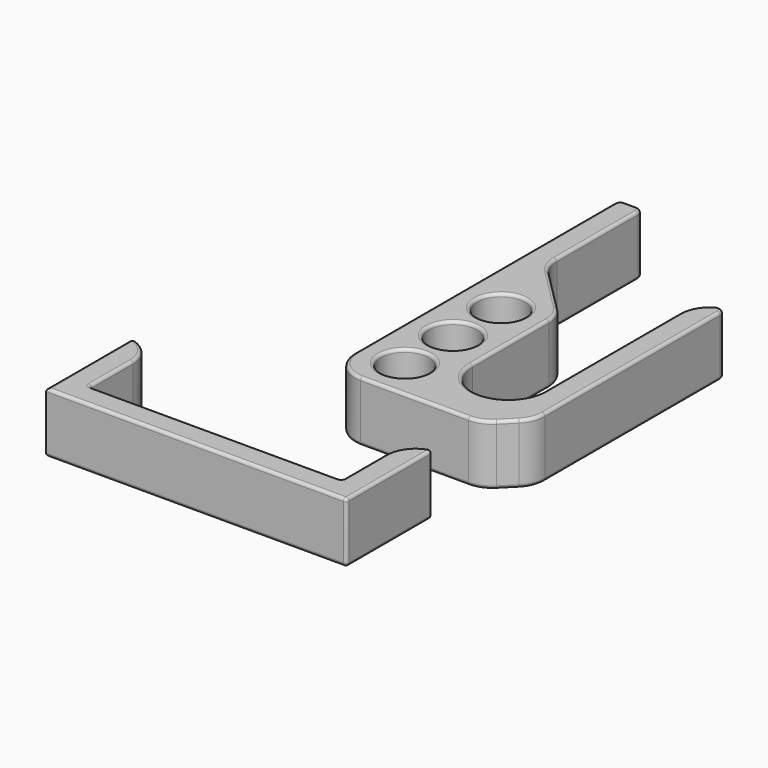
from build123d import *

# Parameters (mm, degrees)
F1_DEPTH     = 10
F2_T1_DEPTH  = 10
F2_T3_DEPTH  = 34.4948974279
F2_T5_DEPTH  = 20.3553390593
F2_T7_DEPTH  = 35
F2_T9_DEPTH  = 20.3553390593
F2_T11_DEPTH = 20.3553390593
F3_R         = 1
F4_R         = 4
F5_DEPTH     = 25
F7_R         = 0.5
F9_DEPTH     = 10
F10_T1_DEPTH = 34.4948974279
F11_R        = 0.5


# Not quite as in the source:
# - a fillet or chamfer that OpenCascade refuses, or shapes differently, is made with other operations: its cross-section is extruded or revolved along the edge and cut away or added
# - a feature names something its author has since deleted; it is built from what else it names


with BuildPart() as f1:
    # F0 (on Top) → F1 (new body)
    with BuildSketch(Plane.XY):
        with BuildLine():
            Line((4, 35.789473919), (0, 35.789473919))
            Line((0, 35.789473919), (0, -24.210526081))
            Line((0, -24.210526081), (25, -24.210526081))
            Line((25, -24.210526081), (30, -19.210526081))
            Line((30, -19.210526081), (30, 20.789473919))
            Line((30, 20.789473919), (26, 20.789473919))
            Line((26, 20.789473919), (26, -12.210526081))
            ThreePointArc((26, -12.210526081), (20, -18.210526081), (14, -12.210526081))
            Line((14, -12.210526081), (14, 5.789473919))
            Line((14, 5.789473919), (4, 15.789473919))
            Line((4, 15.789473919), (4, 35.789473919))
        make_face()
    extrude(amount=F1_DEPTH)

    # F2: fillet of radius 5 on 6 edges, made by hand

    # F2_s2 → F2_t1 (join)
    with BuildSketch(Plane.XY):
        with BuildLine():
            ThreePointArc((5.4644660941, 14.325007825), (4.3806023374, 15.9471245691), (4, 17.8605417309))
            Line((4, 17.8605417309), (4, 15.789473919))
            Line((4, 15.789473919), (5.4644660941, 14.325007825))
        make_face()
    extrude(amount=F2_T1_DEPTH)

    # F2_s4 → F2_t3 (cut)
    with BuildSketch(Plane.XY.offset(-12.2474487139)):
        with BuildLine():
            ThreePointArc((26, 15.8904944335), (27.1270166538, 19.0527720936), (30, 20.789473919))
            Line((30, 20.789473919), (26, 20.789473919))
            Line((26, 20.789473919), (26, 15.8904944335))
        make_face()
    extrude(amount=F2_T3_DEPTH, mode=Mode.SUBTRACT)

    # F2_s6 → F2_t5 (cut)
    with BuildSketch(Plane.XY.offset(-5.1776695297)):
        with BuildLine():
            ThreePointArc((12.5355339059, 7.2539400131), (13.6193976626, 5.631823269), (14, 3.7184061072))
            Line((14, 3.7184061072), (14, 5.789473919))
            Line((14, 5.789473919), (12.5355339059, 7.2539400131))
        make_face()
    extrude(amount=F2_T5_DEPTH, mode=Mode.SUBTRACT)

    # F2_s8 → F2_t7 (cut)
    with BuildSketch(Plane.XY.offset(-12.5)):
        with BuildLine():
            ThreePointArc((5, -24.210526081), (1.4644660941, -22.7460599869), (0, -19.210526081))
            Line((0, -19.210526081), (0, -24.210526081))
            Line((0, -24.210526081), (5, -24.210526081))
        make_face()
    extrude(amount=F2_T7_DEPTH, mode=Mode.SUBTRACT)

    # F2_s10 → F2_t9 (cut)
    with BuildSketch(Plane.XY.offset(-5.1776695297)):
        with BuildLine():
            ThreePointArc((26.4644660941, -22.7460599869), (24.84234935, -23.8299237435), (22.9289321881, -24.210526081))
            Line((22.9289321881, -24.210526081), (25, -24.210526081))
            Line((25, -24.210526081), (26.4644660941, -22.7460599869))
        make_face()
    extrude(amount=F2_T9_DEPTH, mode=Mode.SUBTRACT)

    # F2_s12 → F2_t11 (cut)
    with BuildSketch(Plane.XY.offset(-5.1776695297)):
        with BuildLine():
            ThreePointArc((30, -17.1394582691), (29.6193976626, -19.0528754309), (28.5355339059, -20.674992175))
            Line((28.5355339059, -20.674992175), (30, -19.210526081))
            Line((30, -19.210526081), (30, -17.1394582691))
        make_face()
    extrude(amount=F2_T11_DEPTH, mode=Mode.SUBTRACT)

    # F3
    f3_edges = [f1.edges().sort_by_distance(p)[0] for p in [
        (30, 20.789474, 5),
        (0, 35.789474, 5),
        (4, 35.789474, 5),
    ]]
    fillet(f3_edges, radius=F3_R)


with BuildPart() as f5:
    # F4 (on Top) → F5 (new body)
    with BuildSketch(Plane.XY):
        with Locations((7, 2.5)):
            Circle(F4_R)
    extrude(amount=F5_DEPTH)


with BuildPart() as f5b:
    # F4 (on Top) → F5, piece 2 (new body)
    with BuildSketch(Plane.XY):
        with Locations((7, -7.5)):
            Circle(F4_R)
    extrude(amount=F5_DEPTH)


with BuildPart() as f5c:
    # F4 (on Top) → F5, piece 3 (new body)
    with BuildSketch(Plane.XY):
        with Locations((7, -17.5)):
            Circle(F4_R)
    extrude(amount=F5_DEPTH)


with BuildPart() as f1_1:
    add(f1.part)

    # F6: cut F5c, F5b, F5
    add(f5c.part, mode=Mode.SUBTRACT)
    add(f5b.part, mode=Mode.SUBTRACT)
    add(f5.part, mode=Mode.SUBTRACT)

    # F7
    f7_edges = [f1_1.edges().sort_by_distance(p)[0] for p in [
        (3, -17.5, 10),
        (3, -7.5, 10),
        (3, 2.5, 10),
        (3, 2.5, 0),
        (3, -7.5, 0),
        (3, -17.5, 0),
        (26.669873, 18.390494, 0),
        (29.5, 20.220621, 0),
        (26, 1.839984, 0),
        (30, 1.107569, 0),
        (20, -18.210526, 0),
        (29.619398, -19.052875, 0),
        (14, -4.24606, 0),
        (27.5, -21.710526, 0),
        (13.619398, 5.631823, 0),
        (24.842349, -23.829924, 0),
        (9, 10.789474, 0),
        (13.964466, -24.210526, 0),
        (4.380602, 15.947125, 0),
        (1.464466, -22.74606, 0),
        (4, 26.325008, 0),
        (0, 7.789474, 0),
        (3.707107, 35.496581, 0),
        (0.292893, 35.496581, 0),
        (2, 35.789474, 0),
        (26.669873, 18.390494, 10),
        (29.5, 20.220621, 10),
        (26, 1.839984, 10),
        (30, 1.107569, 10),
        (20, -18.210526, 10),
        (29.619398, -19.052875, 10),
        (14, -4.24606, 10),
        (27.5, -21.710526, 10),
        (13.619398, 5.631823, 10),
        (24.842349, -23.829924, 10),
        (9, 10.789474, 10),
        (13.964466, -24.210526, 10),
        (4.380602, 15.947125, 10),
        (1.464466, -22.74606, 10),
        (4, 26.325008, 10),
        (0, 7.789474, 10),
        (3.707107, 35.496581, 10),
        (0.292893, 35.496581, 10),
        (2, 35.789474, 10),
    ]]
    fillet(f7_edges, radius=F7_R)


with BuildPart() as f9:
    # F8 (on Top) → F9 (new body)
    with BuildSketch(Plane.XY):
        Polygon((-21, -34.1406405903), (-25, -34.1406405903), (-25, -52.1406405903), (25, -52.1406405903), (25, -34.1406405903), (21, -34.1406405903), (21, -48.1406405903), (-21, -48.1406405903), align=None)
    extrude(amount=F9_DEPTH)

    # F10: fillet of radius 5 on 2 edges, made by hand

    # F10_s2 → F10_t1 (cut)
    with BuildSketch(Plane.XY.offset(-12.2474487139)):
        with BuildLine():
            ThreePointArc((25, -34.1406405903), (22.1270166538, -35.8773424157), (21, -39.0396200759))
            Line((21, -39.0396200759), (21, -34.1406405903))
            Line((21, -34.1406405903), (25, -34.1406405903))
        make_face()
        with BuildLine():
            ThreePointArc((-25, -34.1406405903), (-22.1270166538, -35.8773424157), (-21, -39.0396200759))
            Line((-21, -39.0396200759), (-21, -34.1406405903))
            Line((-21, -34.1406405903), (-25, -34.1406405903))
        make_face()
    extrude(amount=F10_T1_DEPTH, mode=Mode.SUBTRACT)

    # F11
    f11_edges = [f9.edges().sort_by_distance(p)[0] for p in [
        (25, -52.140641, 5),
        (25, -34.140641, 5),
        (-25, -34.140641, 5),
        (0, -48.140641, 10),
        (0, -48.140641, 0),
        (-22.127017, -35.877342, 10),
        (-21, -43.59013, 10),
        (21, -43.59013, 10),
        (22.127017, -35.877342, 10),
        (25, -43.140641, 10),
        (0, -52.140641, 10),
        (-25, -43.140641, 10),
        (-22.127017, -35.877342, 0),
        (-21, -43.59013, 0),
        (21, -43.59013, 0),
        (22.127017, -35.877342, 0),
        (25, -43.140641, 0),
        (0, -52.140641, 0),
        (-25, -43.140641, 0),
        (-21, -48.140641, 5),
        (21, -48.140641, 5),
    ]]
    fillet(f11_edges, radius=F11_R)


solid = Compound([f1_1.part, f9.part])
